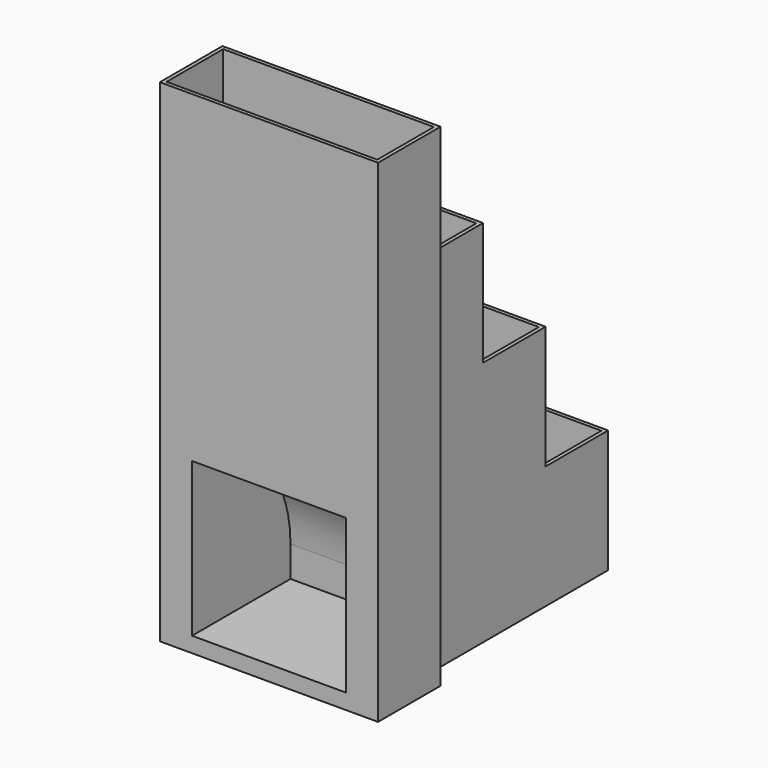
from build123d import *

# Parameters (mm, degrees)
F1_DEPTH      = 57.9
F2_DEPTH      = 64.4
F2_DEPTH_BACK = 6.5
F3_W          = 55.5
F3_H          = 23
F4_DEPTH      = 207
F5_DEPTH      = 116
F6_DEPTH      = 96
F3_W_2        = 68.5
F7_DEPTH      = 39
F8_W          = 50
F8_H          = 50
F9_DEPTH      = 40
F10_R         = 39.99999


# Not quite as in the source:
# - a fillet or chamfer is up to 0.001 mm smaller than in the source, because OpenCascade refuses the exact size


with BuildPart() as f1:
    # F0 (on Right) → F1 (new body)
    with BuildSketch(Plane.YZ):
        Polygon((-124.7912996866, 120), (-124.7912996866, 0), (-48.5912996866, 0), (-48.5912996866, 40), (-73.9912996866, 40), (-73.9912996866, 80), (-99.3912996866, 80), (-99.3912996866, 120), align=None)
    extrude(amount=F1_DEPTH)

    # F0 (on Right) → F2 (join, two sides)
    with BuildSketch(Plane.YZ) as f2_sk:
        Polygon((-150.1912996866, 160), (-150.1912996866, 0), (-124.7912996866, 0), (-124.7912996866, 120), (-124.7912996866, 160), align=None)
    extrude(amount=F2_DEPTH)
    extrude(f2_sk.sketch, amount=-F2_DEPTH_BACK)

    # F3 (on face) → F4 (cut)
    with BuildSketch(Plane.XY.offset(160)):
        with Locations((28.95, -61.2912996866)):
            Rectangle(F3_W, F3_H)
    extrude(amount=-F4_DEPTH, mode=Mode.SUBTRACT)

    # F3 (on face) → F5 (cut, through all)
    with BuildSketch(Plane.XY.offset(160)):
        with Locations((28.95, -86.6912996866)):
            Rectangle(F3_W, F3_H)
    extrude(amount=-F5_DEPTH, mode=Mode.SUBTRACT)

    # F3 (on face) → F6 (cut, through all)
    with BuildSketch(Plane.XY.offset(160)):
        with Locations((28.95, -112.0912996866)):
            Rectangle(F3_W, F3_H)
    extrude(amount=-F6_DEPTH, mode=Mode.SUBTRACT)

    # F3 (on face) → F7 (cut)
    with BuildSketch(Plane.XY.offset(160)):
        with Locations((28.95, -137.4912996866)):
            Rectangle(F3_W_2, F3_H)
    extrude(amount=-F7_DEPTH, mode=Mode.SUBTRACT)

    # F8 (on face) → F9 (cut)
    with BuildSketch(Plane.XZ.offset(150.1912996866)):
        with Locations((28.95, 30)):
            Rectangle(F8_W, F8_H)
    extrude(amount=-F9_DEPTH, mode=Mode.SUBTRACT)

    # F10 (radius 40 in the source; OpenCascade refuses exactly that, so slightly less here)
    f10_edges = [f1.edges().sort_by_distance(p)[0] for p in [
        (28.95, -110.1913, 55),
    ]]
    fillet(f10_edges, radius=F10_R)


solid = f1.part
